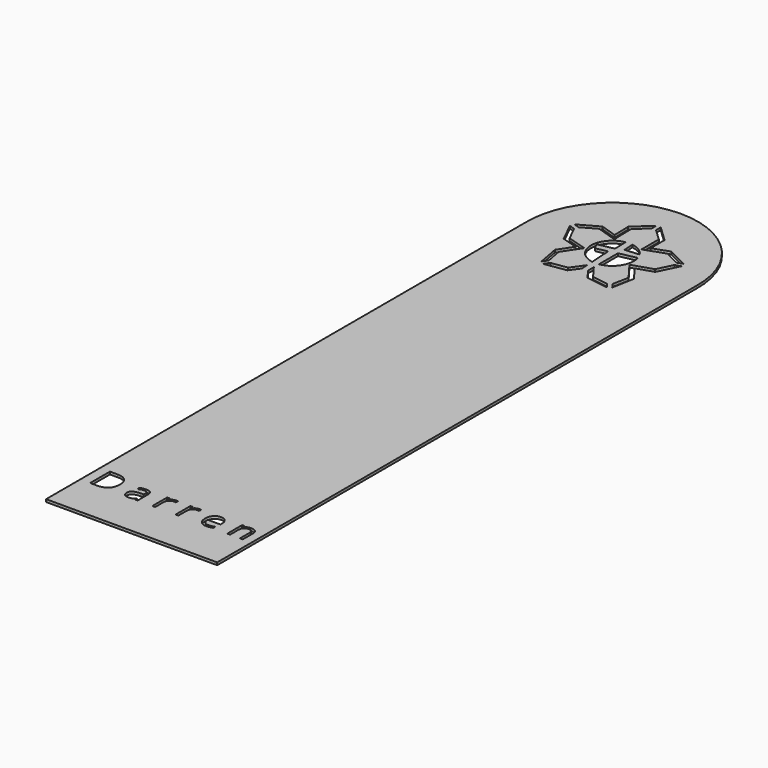
from build123d import *

# Parameters (mm, degrees)
F1_DEPTH     = 0.6
F2_TEXT_SIZE = 8.1116299469
F3_DEPTH     = 25


# Not quite as in the source:
# - Text() gives the source's letters only with a copy of the font that has no kerning and outlines rounded to 1/6400 em; it was checked with that copy


with BuildPart() as f1:
    # F0 (on Top) → F1 (new body)
    with BuildSketch(Plane.XY):
        with BuildLine():
            Line((-6.2929817945, -85.9107411313), (-6.2929817945, 54.0892588687))
            ThreePointArc((-6.2929817945, 54.0892588687), (-26.2881293893, 74.529795656), (-46.2832769841, 54.0892588687))
            Line((-46.2832769841, 54.0892588687), (-46.2832769841, -85.9107411313))
            Line((-46.2832769841, -85.9107411313), (-6.2929817945, -85.9107411313))
        make_face()
        Polygon((-39.1357927602, 58.156282706), (-37.8167754178, 57.7488087208), (-36.0964508727, 54.2858152185), (-31.5504507998, 52.9304291024), (-34.2764975503, 48.8383139018), (-33.5787166392, 45.068726519), (-34.3857806482, 43.9346634595), (-35.333623671, 49.0551490486), (-33.1328767374, 52.3587277484), (-36.798669675, 53.4516808439), align=None, mode=Mode.SUBTRACT)
        Polygon((-33.5710354633, 43.3548442777), (-32.7639714543, 44.4889073372), (-29.0395161137, 45.0546483044), (-26.9457103872, 47.9622273289), (-26.8474352261, 46.3874498879), (-28.4737006293, 44.1291242395), align=None, mode=Mode.SUBTRACT)
        Polygon((-29.5887580141, 64.1036548186), (-29.4783906855, 59.0562246323), (-34.1743482277, 60.578727629), (-37.5216161236, 58.7042567785), (-38.840633466, 59.1117307637), (-34.2816513675, 61.6647618677), (-30.5089220455, 60.4415839222), (-30.598373451, 64.5324659769), (-26.7969193064, 68.043156412), (-26.8055869837, 66.6739480655), align=None, mode=Mode.SUBTRACT)
        with BuildLine():
            Line((-30.0487077198, 54.0772011169), (-27.3612933233, 54.6215970535))
            Line((-27.3612933233, 54.6215970535), (-27.0471519031, 49.5877429627))
            ThreePointArc((-27.0471519031, 49.5877429627), (-31.2879394854, 54.4862181068), (-27.1331783382, 59.4578675177))
            Line((-27.1331783382, 59.4578675177), (-27.0563370558, 56.2451489523))
            Line((-27.0563370558, 56.2451489523), (-30.742992647, 55.4983343463))
            Line((-30.742992647, 55.4983343463), (-30.0487077198, 54.0772011169))
        make_face(mode=Mode.SUBTRACT)
        Polygon((-25.4982272163, 46.435824232), (-25.4982272163, 48.115820707), (-23.2306225225, 45.0546483044), (-19.4864443863, 44.4883009736), (-18.6820422025, 43.3552512513), (-23.7884122058, 44.1276447957), align=None, mode=Mode.SUBTRACT)
        with BuildLine():
            Line((-25.4982272163, 49.5925844435), (-25.4982272163, 55.1695583854))
            Line((-25.4982272163, 55.1695583854), (-21.5027353554, 55.9789346902))
            ThreePointArc((-21.5027353554, 55.9789346902), (-22.0493383686, 51.8778811244), (-25.4982272163, 49.5925844435))
        make_face(mode=Mode.SUBTRACT)
        Polygon((-17.8666377764, 43.9341429699), (-18.6710399602, 45.0671926922), (-17.9616594687, 48.8383139018), (-21.0258079788, 52.9304291024), (-16.2674002349, 54.4754809234), (-14.5643813054, 57.960361879), (-13.2345696342, 58.4039797299), (-15.5551681686, 53.6553480512), (-19.3875651028, 52.4109713225), (-16.8975931641, 49.0856586015), align=None, mode=Mode.SUBTRACT)
        with BuildLine():
            Line((-22.0889890684, 57.2440580909), (-25.3886347637, 56.9700004999))
            Line((-25.3886347637, 56.9700004999), (-25.5972594206, 59.481835507))
            ThreePointArc((-25.5972594206, 59.481835507), (-23.5992705051, 58.7452479332), (-22.0889890684, 57.2440580909))
        make_face(mode=Mode.SUBTRACT)
        Polygon((-13.5510203564, 59.3525886801), (-14.8808320276, 58.9089708292), (-18.3619530872, 60.6872062199), (-23.0988633455, 59.0107087439), (-23.0988633455, 64.1036548186), (-25.8056070202, 66.6676177626), (-25.796939343, 68.0368261091), (-22.0988633455, 64.5338236232), (-22.0988633455, 60.4254140461), (-18.2901023062, 61.7734189524), align=None, mode=Mode.SUBTRACT)
    extrude(amount=F1_DEPTH)

    # F2 (on face) → F3 (cut)
    with BuildSketch(Plane.XY.offset(0.6)):
        with BuildLine():
            add(Edge.make_bspline(
                [(-40.6837352555, -74.7364559523), (-40.0772641727, -74.1439267335), (-40.0772641727, -72.9842171396)],
                knots=[0, 0, 0, 1, 1, 1], degree=2))
            add(Edge.make_bspline(
                [(-40.0772641727, -72.9842171396), (-40.0772641727, -71.8511238313), (-40.6457119901, -71.2769725242)],
                knots=[0, 0, 0, 1, 1, 1], degree=2))
            add(Edge.make_bspline(
                [(-40.6457119901, -71.2769725242), (-41.2141598075, -70.702821217), (-42.3358461361, -70.702821217)],
                knots=[0, 0, 0, 1, 1, 1], degree=2))
            Line((-42.3358461361, -70.702821217), (-43.3143114984, -70.702821217))
            Line((-43.3143114984, -70.702821217), (-43.3143114984, -75.3289851711))
            Line((-43.3143114984, -75.3289851711), (-42.4942764085, -75.3289851711))
            add(Edge.make_bspline(
                [(-42.4942764085, -75.3289851711), (-41.2902063382, -75.3289851711), (-40.6837352555, -74.7364559523)],
                knots=[0, 0, 0, 1, 1, 1], degree=2))
        make_face()
        with Locations((-44.7832769841, -75.9107411313)):
            Text('D a r r e n', F2_TEXT_SIZE, font='Open Sans', text_align=(TextAlign.LEFT, TextAlign.BOTTOM))
        with BuildLine():
            add(Edge.make_bspline(
                [(-35.4840537153, -75.2611770145), (-35.2685885448, -75.4468572937), (-34.880751238, -75.4468572937)],
                knots=[0, 0, 0, 1, 1, 1], degree=2))
            add(Edge.make_bspline(
                [(-34.880751238, -75.4468572937), (-34.2660417811, -75.4468572937), (-33.9155940186, -75.1103513952)],
                knots=[0, 0, 0, 1, 1, 1], degree=2))
            add(Edge.make_bspline(
                [(-33.9155940186, -75.1103513952), (-33.565146256, -74.7738454966), (-33.565146256, -74.1680081349)],
                knots=[0, 0, 0, 1, 1, 1], degree=2))
            Line((-33.565146256, -74.1680081349), (-33.565146256, -73.7763685016))
            Line((-33.565146256, -73.7763685016), (-34.222948747, -73.8029847873))
            add(Edge.make_bspline(
                [(-34.222948747, -73.8029847873), (-35.0074954559, -73.8308685153), (-35.3535071709, -74.0469674068)],
                knots=[0, 0, 0, 1, 1, 1], degree=2))
            add(Edge.make_bspline(
                [(-35.3535071709, -74.0469674068), (-35.6995188858, -74.2630662984), (-35.6995188858, -74.7180780407)],
                knots=[0, 0, 0, 1, 1, 1], degree=2))
            add(Edge.make_bspline(
                [(-35.6995188858, -74.7180780407), (-35.6995188858, -75.0754967352), (-35.4840537153, -75.2611770145)],
                knots=[0, 0, 0, 1, 1, 1], degree=2))
        make_face()
        with BuildLine():
            add(Edge.make_bspline(
                [(-16.1587290879, -72.372042567), (-16.4356652041, -72.0412401582), (-16.951514171, -72.0412401582)],
                knots=[0, 0, 0, 1, 1, 1], degree=2))
            add(Edge.make_bspline(
                [(-16.951514171, -72.0412401582), (-17.4737003489, -72.0412401582), (-17.7848574039, -72.3815483833)],
                knots=[0, 0, 0, 1, 1, 1], degree=2))
            add(Edge.make_bspline(
                [(-17.7848574039, -72.3815483833), (-18.0960144588, -72.7218566085), (-18.1517819147, -73.3238916436)],
                knots=[0, 0, 0, 1, 1, 1], degree=2))
            Line((-18.1517819147, -73.3238916436), (-15.8817929718, -73.3238916436))
            add(Edge.make_bspline(
                [(-15.8817929718, -73.3238916436), (-15.8817929718, -72.7028449758), (-16.1587290879, -72.372042567)],
                knots=[0, 0, 0, 1, 1, 1], degree=2))
        make_face()
    extrude(amount=-F3_DEPTH, mode=Mode.SUBTRACT)


solid = f1.part
